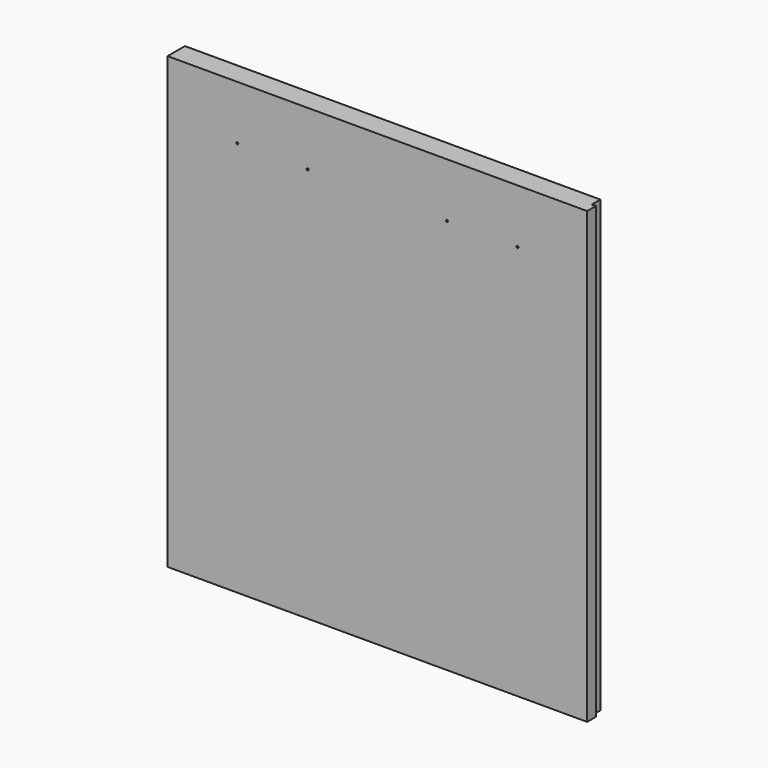
from build123d import *

# Parameters (mm, degrees)
F0_W           = 1966.9125
F0_H           = 2108.2
F1_DEPTH       = 101.6
F2_W           = 19.05
F2_H           = 50.8
F3_DEPTH       = 2108.201
F6_D           = 9.525
F6_CSINK_D     = 19.8374
F6_CSINK_ANGLE = 82


# Not quite as in the source:
# - a feature names something its author has since deleted; it is built from what else it names


with BuildPart() as f1:
    # F0 (on Front) → F1 (new body)
    with BuildSketch(Plane.XZ):
        with Locations((983.45625, 1054.1)):
            Rectangle(F0_W, F0_H)
    extrude(amount=F1_DEPTH)

    # F2 (on face) → F3 (cut, through all)
    with BuildSketch(Plane.XY.offset(2108.2)):
        with Locations((1957.3875, -25.4)):
            Rectangle(F2_W, F2_H)
    extrude(amount=-F3_DEPTH, mode=Mode.SUBTRACT)

    # F6 (through all)
    with Locations(Plane(origin=(0, 0, 0), x_dir=(-1, 0, 0), z_dir=(0, 1, 0))):
        with Locations((-1640.284375, 1854.2), (-1310.084375, 1854.2), (-656.828125, 1854.2), (-326.628125, 1854.2)):
            CounterSinkHole(F6_D / 2, F6_CSINK_D / 2, counter_sink_angle=F6_CSINK_ANGLE)


solid = f1.part
